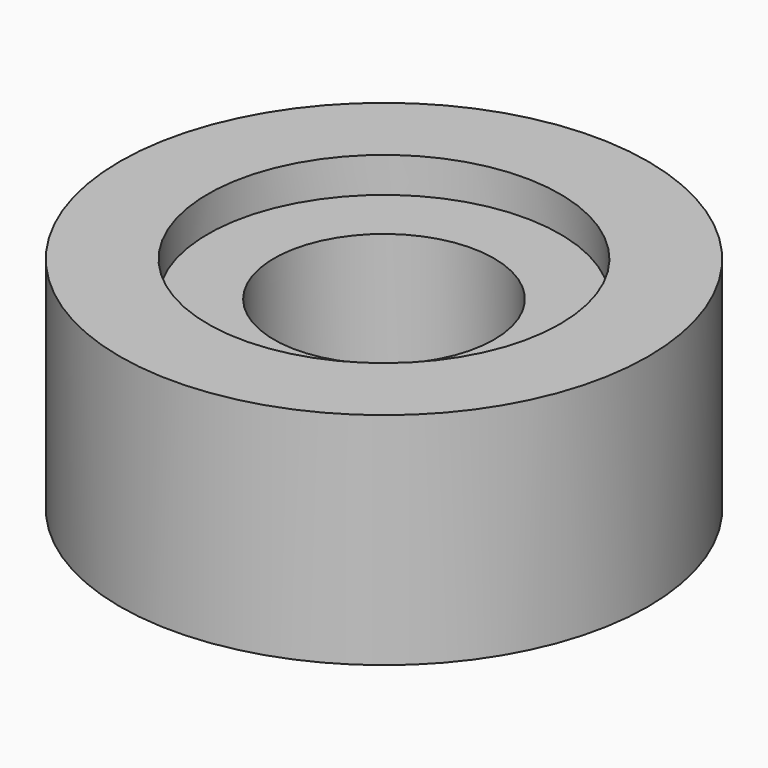
from build123d import *

# Parameters (mm, degrees)
F0_R     = 9.525
F0_R_2   = 6.35
F0_R_3   = 3.96875
F1_DEPTH = 7.9375
F2_DEPTH = 1.27


# Not quite as in the source:
# - a length typed as a fraction of an inch, garbled in the dataset ("3 / 203.2 mm" for 3/8 in), is restored


with BuildPart() as f1:
    # F0 (on Top) → F1 (new body)
    with BuildSketch(Plane.XY):
        Circle(F0_R)
        Circle(F0_R_2, mode=Mode.SUBTRACT)
        Circle(F0_R_2)
        Circle(F0_R_3, mode=Mode.SUBTRACT)
    extrude(amount=-F1_DEPTH)

    # F0 (on Top) → F2 (cut)
    with BuildSketch(Plane.XY):
        Circle(F0_R_2)
        Circle(F0_R_3, mode=Mode.SUBTRACT)
    extrude(amount=-F2_DEPTH, mode=Mode.SUBTRACT)


solid = f1.part
